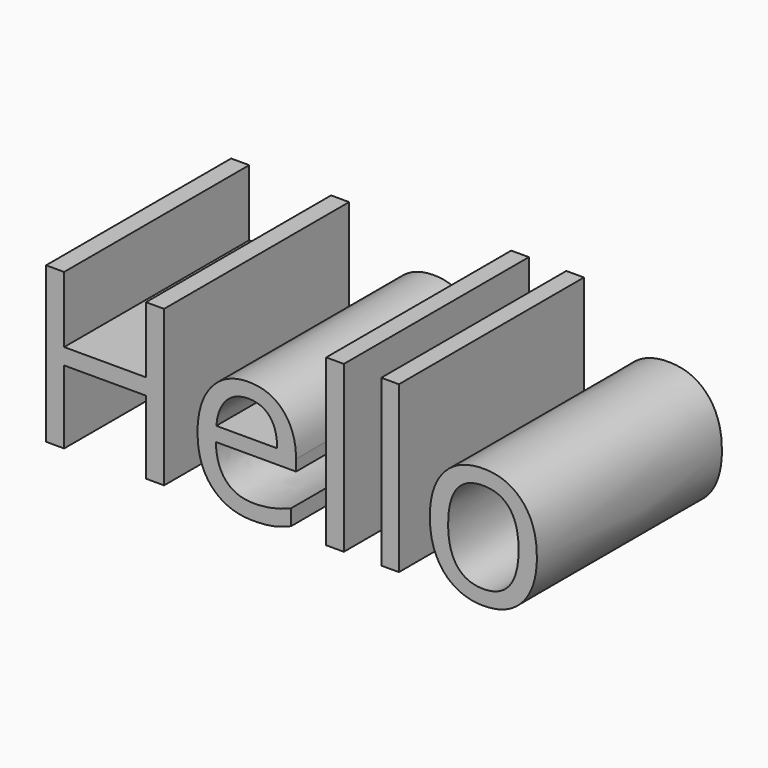
from build123d import *

# Parameters (mm, degrees)
F0_TEXT_SIZE = 23.9047952669
F1_DEPTH     = 25.4


# Not quite as in the source:
# - Text() gives the source's letters only with a copy of the font that has no kerning and outlines rounded to 1/6400 em; it was checked with that copy


with BuildPart() as f1:
    # F0 (on Front) → F1 (new body)
    with BuildSketch(Plane.XZ):
        with Locations((-57.7979236841, 5.465799477)):
            Text('Hello', F0_TEXT_SIZE, font='Open Sans', text_align=(TextAlign.LEFT, TextAlign.BOTTOM))
    extrude(amount=F1_DEPTH)


solid = f1.part
